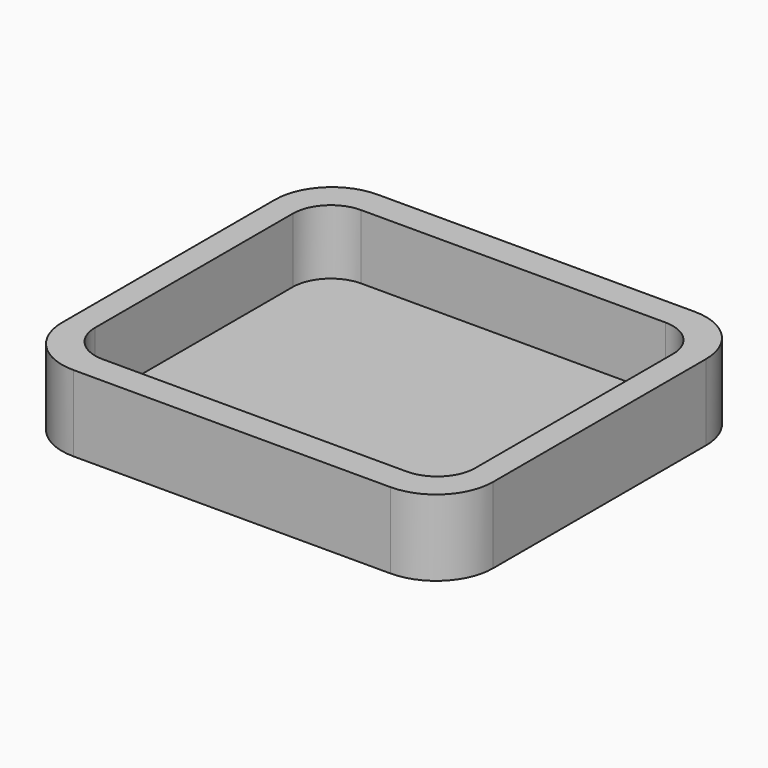
from build123d import *

# Parameters (mm, degrees)
F0_W         = 1134.4351611798
F0_H         = 1000
F1_DEPTH     = 200
F2_R         = 150
F3_W         = 1000
F3_H         = 850
F4_DEPTH     = 170
F5_R         = 100
F6_TEXT_SIZE = 63.0858855188
F7_DEPTH     = 15


# Not quite as in the source:
# - Text() gives the source's letters only with a copy of the font that has no kerning and outlines rounded to 1/6400 em; it was checked with that copy


with BuildPart() as f1:
    # F0 (on Top) → F1 (new body)
    with BuildSketch(Plane.XY):
        Rectangle(F0_W, F0_H)
    extrude(amount=F1_DEPTH)

    # F2
    f2_edges = [f1.edges().sort_by_distance(p)[0] for p in [
        (-567.217581, -500, 100),
        (567.217581, -500, 100),
        (567.217581, 500, 100),
        (-567.217581, 500, 100),
    ]]
    fillet(f2_edges, radius=F2_R)

    # F3 (on face) → F4 (cut)
    with BuildSketch(Plane.XY.offset(200)):
        Rectangle(F3_W, F3_H)
    extrude(amount=-F4_DEPTH, mode=Mode.SUBTRACT)

    # F5
    f5_edges = [f1.edges().sort_by_distance(p)[0] for p in [
        (500, 425, 115),
        (500, -425, 115),
        (-500, 425, 115),
        (-500, -425, 115),
    ]]
    fillet(f5_edges, radius=F5_R)

    # F6 (on face) → F7 (join)
    with BuildSketch(Plane(origin=(0, 0, 0), x_dir=(1, 0, 0), z_dir=(0, 0, -1))):
        with Locations((-504.5848653543, 381.7348297797)):
            Text('Detonador Remoto 18 V Marte 1', F6_TEXT_SIZE, font='Open Sans', font_style=FontStyle.BOLD, text_align=(TextAlign.LEFT, TextAlign.BOTTOM))
    extrude(amount=F7_DEPTH)


solid = f1.part
